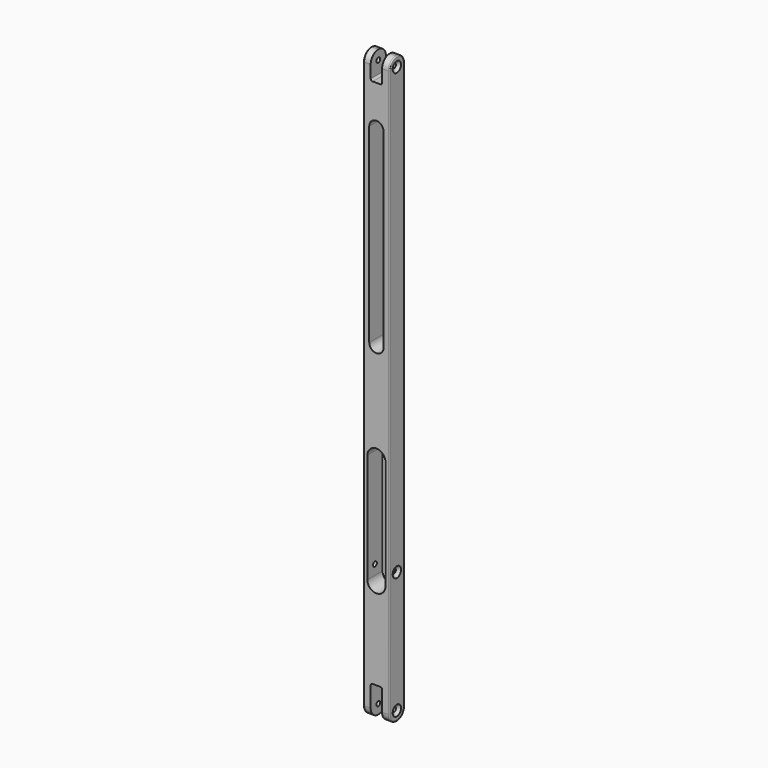
from build123d import *

# Parameters (mm, degrees)
F0_W      = 27
F0_H      = 615
F1_DEPTH  = 20
F2_W      = 12
F2_H      = 20
F3_DEPTH  = 25
F4_W      = 12
F4_H      = 20
F5_DEPTH  = 33
F6_R      = 9.99999
F7_R      = 2.5
F8_DEPTH  = 30
F10_DEPTH = 25
F11_R     = 2.5
F12_DEPTH = 30
F14_DEPTH = 25
F15_R     = 1
F16_SIZE  = 3
F17_R     = 2


# Not quite as in the source:
# - a fillet or chamfer is up to 0.001 mm smaller than in the source, because OpenCascade refuses the exact size


with BuildPart() as f1:
    # F0 (on Front) → F1 (new body)
    with BuildSketch(Plane.XZ):
        Rectangle(F0_W, F0_H)
    extrude(amount=F1_DEPTH)

    # F2 (on face) → F3 (cut)
    with BuildSketch(Plane.XY.offset(307.5)):
        with Locations((0, -10)):
            Rectangle(F2_W, F2_H)
    extrude(amount=-F3_DEPTH, mode=Mode.SUBTRACT)

    # F4 (on face) → F5 (cut)
    with BuildSketch(Plane(origin=(0, 0, -307.5), x_dir=(1, 0, 0), z_dir=(0, 0, -1))):
        with Locations((0, 10)):
            Rectangle(F4_W, F4_H)
    extrude(amount=-F5_DEPTH, mode=Mode.SUBTRACT)

    # F6 (radius 10 in the source; OpenCascade refuses exactly that, so slightly less here)
    f6_edges = [f1.edges().sort_by_distance(p)[0] for p in [
        (-9.75, 0, -307.5),
        (9.75, 0, -307.5),
        (9.75, -20, -307.5),
        (-9.75, -20, -307.5),
        (-9.75, -20, 307.5),
        (-9.75, 0, 307.5),
        (9.75, 0, 307.5),
        (9.75, -20, 307.5),
    ]]
    fillet(f6_edges, radius=F6_R)

    # F7 (on face) → F8 (cut)
    with BuildSketch(Plane(origin=(-13.5, 0, 0), x_dir=(0, -1, 0), z_dir=(-1, 0, 0))):
        with Locations((10, 297.5)):
            Circle(F7_R)
        with Locations((10, -297.5)):
            Circle(F7_R)
    extrude(amount=-F8_DEPTH, mode=Mode.SUBTRACT)

    # F9 (on face) → F10 (cut)
    with BuildSketch(Plane.XZ.offset(20)):
        with BuildLine():
            ThreePointArc((9.5, -65), (0, -55.5), (-9.5, -65))
            Line((-9.5, -65), (-9.5, -180))
            ThreePointArc((-9.5, -180), (0, -189.5), (9.5, -180))
            Line((9.5, -180), (9.5, -65))
        make_face()
    extrude(amount=-F10_DEPTH, mode=Mode.SUBTRACT)

    # F11 (on face) → F12 (cut)
    with BuildSketch(Plane(origin=(-13.5, 0, 0), x_dir=(0, -1, 0), z_dir=(-1, 0, 0))):
        with Locations((10, -169.5)):
            Circle(F11_R)
    extrude(amount=-F12_DEPTH, mode=Mode.SUBTRACT)

    # F13 (on face) → F14 (cut)
    with BuildSketch(Plane.XZ.offset(20)):
        with BuildLine():
            ThreePointArc((7.5, 240), (0, 247.5), (-7.5, 240))
            Line((-7.5, 240), (-7.5, 40))
            ThreePointArc((-7.5, 40), (0, 32.5), (7.5, 40))
            Line((7.5, 40), (7.5, 240))
        make_face()
    extrude(amount=-F14_DEPTH, mode=Mode.SUBTRACT)

    # F15
    f15_edges = [f1.edges().sort_by_distance(p)[0] for p in [
        (13.5, -20, 0),
        (-13.5, -20, 0),
    ]]
    fillet(f15_edges, radius=F15_R)

    # F16
    f16_edges = [f1.edges().sort_by_distance(p)[0] for p in [
        (13.5, -7.5, 297.5),
        (13.5, -7.5, -169.5),
        (13.5, -7.5, -297.5),
    ]]
    chamfer(f16_edges, length=F16_SIZE)

    # F17
    f17_edges = [f1.edges().sort_by_distance(p)[0] for p in [
        (-6, -10, 282.5),
        (6, -10, 282.5),
        (6, -10, -274.5),
        (-6, -10, -274.5),
    ]]
    fillet(f17_edges, radius=F17_R)


solid = f1.part
